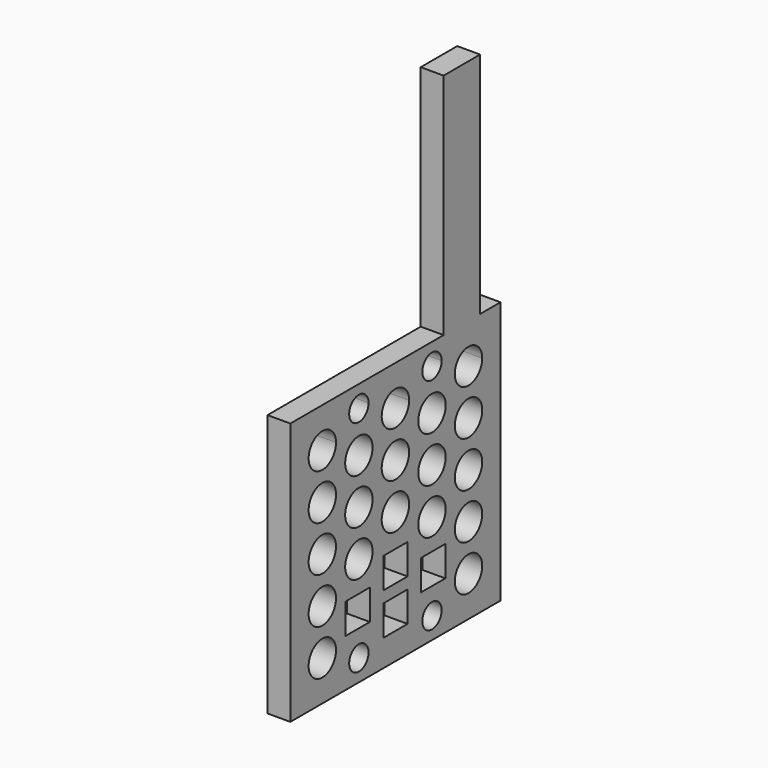
from build123d import *

# Parameters (mm, degrees)
F0_R     = 0.75
F0_R_2   = 0.53
F1_DEPTH = 1


# Not quite as in the source:
# - a feature names something its author has since deleted; it is built from what else it names


with BuildPart() as f1:
    # F0 (on Right) → F1 (new body)
    with BuildSketch(Plane.YZ):
        Polygon((1.75, 0), (0, 0), (0, -11.5), (11.5, -11.5), (11.5, 0), (10.384144865, 0), (10.384144865, 10), (8.384144865, 10), (8.384144865, 0), (7.7499999977, 0), (5.750004947, 0), (3.75, 0), align=None)
        with Locations((1.7500000088, -9.75)):
            Circle(F0_R, mode=Mode.SUBTRACT)
        with Locations((1.75, -7.75)):
            Circle(F0_R, mode=Mode.SUBTRACT)
        with Locations((3.7499851588, -10.5567658602)):
            Circle(F0_R_2, mode=Mode.SUBTRACT)
        Polygon((5.3081902647, -9.0000098941), (5.7499752647, -9.0000098941), (6.1917602647, -9.0000098941), (6.4146452647, -9.0000098941), (6.4146452647, -10.3293498941), (6.1917602647, -10.3293498941), (5.0853052647, -10.3293498941), (5.0853052647, -9.0000098941), align=None, mode=Mode.SUBTRACT)
        Polygon((3.1706485936, -8.0853299912), (4.3492385936, -8.0853299912), (4.3492385936, -8.7499999912), (4.3492385936, -9.4146699912), (3.1706485936, -9.4146699912), (3.0198985936, -9.4146699912), (3.0198985936, -8.7499999912), (3.0198985936, -8.0853299912), align=None, mode=Mode.SUBTRACT)
        with Locations((3.7499923957, -6.75)):
            Circle(F0_R, mode=Mode.SUBTRACT)
        Polygon((6.4146452647, -8.5000098941), (5.7499752647, -8.5000098941), (5.0853052647, -8.5000098941), (5.0853052647, -7.1706698941), (6.1917602647, -7.1706698941), (6.4146452647, -7.1706698941), align=None, mode=Mode.SUBTRACT)
        with Locations((1.75, -5.75)):
            Circle(F0_R, mode=Mode.SUBTRACT)
        with Locations((1.75, -3.75)):
            Circle(F0_R, mode=Mode.SUBTRACT)
        with BuildLine():
            ThreePointArc((2.5, -1.75), (1.2196699141, -2.2803300859), (1.75, -1))
            ThreePointArc((1.75, -1), (2.2803300859, -1.2196699141), (2.5, -1.75))
        make_face(mode=Mode.SUBTRACT)
        with Locations((3.7499961979, -4.75)):
            Circle(F0_R, mode=Mode.SUBTRACT)
        with Locations((5.7499851588, -5.7500098941)):
            Circle(F0_R, mode=Mode.SUBTRACT)
        with Locations((5.7499950529, -3.7500098941)):
            Circle(F0_R, mode=Mode.SUBTRACT)
        with Locations((3.75, -2.75)):
            Circle(F0_R, mode=Mode.SUBTRACT)
        with BuildLine():
            ThreePointArc((4.28, -0.94325), (3.375233406, -1.318016594), (3.75, -0.41325))
            ThreePointArc((3.75, -0.41325), (4.124766594, -0.568483406), (4.28, -0.94325))
        make_face(mode=Mode.SUBTRACT)
        with Locations((7.749955461, -10.5567658602)):
            Circle(F0_R_2, mode=Mode.SUBTRACT)
        Polygon((7.1507119358, -8.7499999912), (7.1507119358, -8.0853299912), (8.3293019358, -8.0853299912), (8.4800519358, -8.0853299912), (8.4800519358, -8.7499999912), (8.4800519358, -9.4146699912), (8.3293019358, -9.4146699912), (7.1507119358, -9.4146699912), align=None, mode=Mode.SUBTRACT)
        with Locations((7.7499680167, -6.7500197925)):
            Circle(F0_R, mode=Mode.SUBTRACT)
        with Locations((9.7499307145, -9.750039585)):
            Circle(F0_R, mode=Mode.SUBTRACT)
        with Locations((9.749950516, -7.7500395851)):
            Circle(F0_R, mode=Mode.SUBTRACT)
        with Locations((7.7499840072, -4.7500197926)):
            Circle(F0_R, mode=Mode.SUBTRACT)
        with BuildLine():
            ThreePointArc((6.500004947, -1.7500098941), (5.2196748611, -2.28033998), (5.750004947, -1.0000098941))
            ThreePointArc((5.750004947, -1.0000098941), (6.2803350329, -1.2196798082), (6.500004947, -1.7500098941))
        make_face(mode=Mode.SUBTRACT)
        with Locations((7.7499999977, -2.7500197927)):
            Circle(F0_R, mode=Mode.SUBTRACT)
        with BuildLine():
            ThreePointArc((8.2799999977, -0.9432697927), (7.3752334037, -1.3180363867), (7.7499999977, -0.4132697927))
            ThreePointArc((7.7499999977, -0.4132697927), (8.1247665918, -0.5685031986), (8.2799999977, -0.9432697927))
        make_face(mode=Mode.SUBTRACT)
        with Locations((9.7499703087, -5.7500395852)):
            Circle(F0_R, mode=Mode.SUBTRACT)
        with Locations((9.7499901013, -3.7500395853)):
            Circle(F0_R, mode=Mode.SUBTRACT)
        with BuildLine():
            ThreePointArc((9.750009894, -1.0000395854), (10.2803399799, -1.2197094995), (10.500009894, -1.7500395854))
            ThreePointArc((10.500009894, -1.7500395854), (9.2196798081, -2.2803696712), (9.750009894, -1.0000395854))
        make_face(mode=Mode.SUBTRACT)
    extrude(amount=F1_DEPTH)


solid = f1.part
